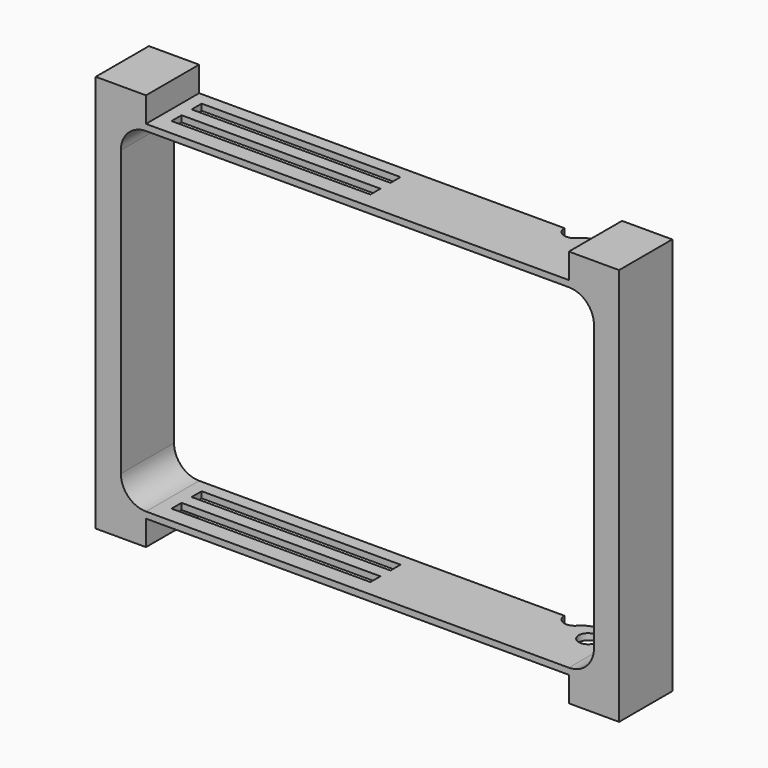
from build123d import *

# Parameters (mm, degrees)
F0_W      = 113
F0_H      = 80
F1_DEPTH  = 15.875
F2_R      = 6
F3_W      = 89
F3_H      = 3
F3_W_2    = 95
F3_R      = 1.5
F4_DEPTH  = 132
F5_W      = 42.9403819144
F5_H      = 7.4070980772
F6_DEPTH  = 1.5
F7_W      = 42.8083911538
F7_H      = 7.2430414148
F8_DEPTH  = 1.5
F9_R      = 2.5
F10_DEPTH = 92
F11_R     = 2.25
F12_DEPTH = 200
F13_R     = 5


with BuildPart() as f1:
    # F0 (on Front) → F1 (new body)
    with BuildSketch(Plane.XZ):
        Polygon((-50.5, 47.5), (-62.5, 47.5), (-62.5, -47.5), (-50.5, -47.5), (-50.5, -41.5), (50.5, -41.5), (50.5, -47.5), (62.5, -47.5), (62.5, 47.5), (50.5, 47.5), (50.5, 41.5), (-50.5, 41.5), align=None)
        Rectangle(F0_W, F0_H, mode=Mode.SUBTRACT)
    extrude(amount=F1_DEPTH)

    # F2
    f2_edges = [f1.edges().sort_by_distance(p)[0] for p in [
        (56.5, -7.9375, 40),
        (56.5, -7.9375, -40),
        (-56.5, -7.9375, -40),
        (-56.5, -7.9375, 40),
    ]]
    fillet(f2_edges, radius=F2_R)

    # F3 (on face) → F4 (cut)
    with BuildSketch(Plane.XY.offset(41.5)):
        with Locations((-3, -4.5)):
            Rectangle(F3_W, F3_H)
        with Locations((0, -10.5)):
            Rectangle(F3_W_2, F3_H)
        with Locations((46, -4.5)):
            Circle(F3_R)
    extrude(amount=-F4_DEPTH, mode=Mode.SUBTRACT)

    # F5 (on face) → F6 (join)
    with BuildSketch(Plane.XY.offset(41.5)):
        with Locations((21.4701909572, -3.7035490386)):
            Rectangle(F5_W, F5_H)
        Polygon((42.9403819144, -7.4070980772), (0, -7.4070980772), (0, -14.1382440925), (49.1435937583, -14.1382440925), (49.1435937583, -7.4070980772), align=None)
    extrude(amount=-F6_DEPTH)

    # F7 (on face) → F8 (join)
    with BuildSketch(Plane(origin=(0, 0, -41.5), x_dir=(1, 0, 0), z_dir=(0, 0, -1))):
        Polygon((49.0116067231, 15.875), (0, 15.875), (0, 7.2430414148), (42.8083911538, 7.2430414148), (49.0116067231, 7.2430414148), align=None)
        with Locations((21.4041955769, 3.6215207074)):
            Rectangle(F7_W, F7_H)
    extrude(amount=-F8_DEPTH)

    # F9 (on face) → F10 (cut)
    with BuildSketch(Plane.XY.offset(41.5)):
        with Locations((39.25, 0)):
            Circle(F9_R)
    extrude(amount=-F10_DEPTH, mode=Mode.SUBTRACT)

    # F11 (on face) → F12 (cut)
    with BuildSketch(Plane.XY.offset(41.5)):
        with Locations((46, -4.5)):
            Circle(F11_R)
    extrude(amount=-F12_DEPTH, mode=Mode.SUBTRACT)

    # F13
    f13_edges = [f1.edges().sort_by_distance(p)[0] for p in [
        (41.75, 0, 40.75),
        (41.75, 0, -40.75),
    ]]
    fillet(f13_edges, radius=F13_R)


solid = f1.part
